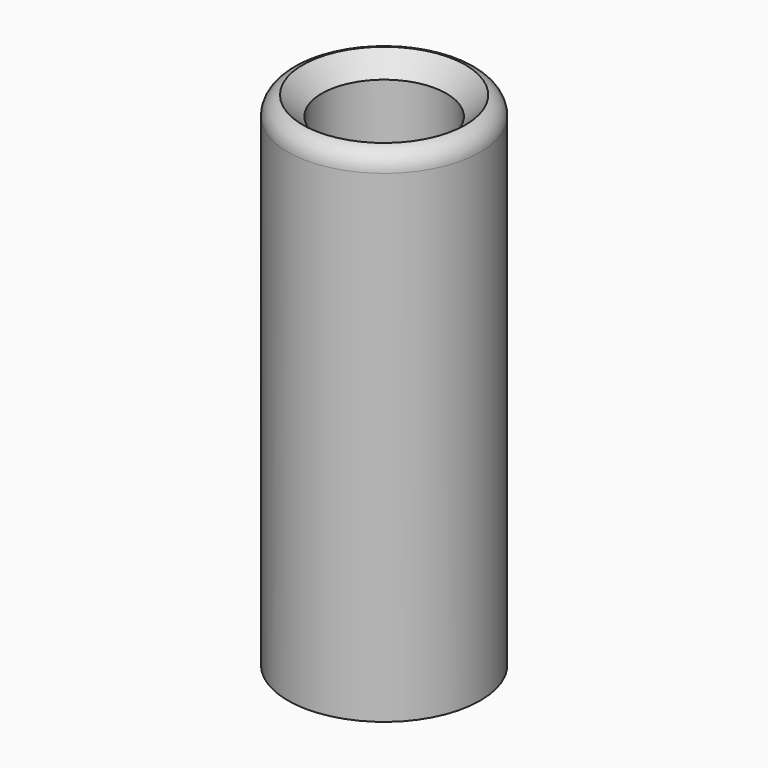
from build123d import *

# Parameters (mm, degrees)
F0_R     = 14.75
F1_DEPTH = 77
F2_R     = 9.55
F3_DEPTH = 77.001
F4_R     = 3


# Not quite as in the source:
# - a fillet or chamfer that OpenCascade refuses, or shapes differently, is made with other operations: its cross-section is extruded or revolved along the edge and cut away or added


with BuildPart() as f1:
    # F0 (on Top) → F1 (new body)
    with BuildSketch(Plane.XY):
        Circle(F0_R)
    extrude(amount=F1_DEPTH)

    # F2 (on Top) → F3 (cut, through all)
    with BuildSketch(Plane.XY):
        Circle(F2_R)
    extrude(amount=F3_DEPTH, mode=Mode.SUBTRACT)

    # F4
    f4_edges = [f1.edges().sort_by_distance(p)[0] for p in [
        (-14.75, 0, 77),
    ]]
    fillet(f4_edges, radius=F4_R)

    # F5: chamfer of 3 on 1 edges, made by hand

    # F5_s1 → F5_t2 (revolve, cut)
    with BuildSketch(Plane.XZ):
        Polygon((12.55, 77), (9.55, 74), (9.55, 77), align=None)
    revolve(axis=Axis((0, 0, 77), (0, 0, -1)), mode=Mode.SUBTRACT)


solid = f1.part
